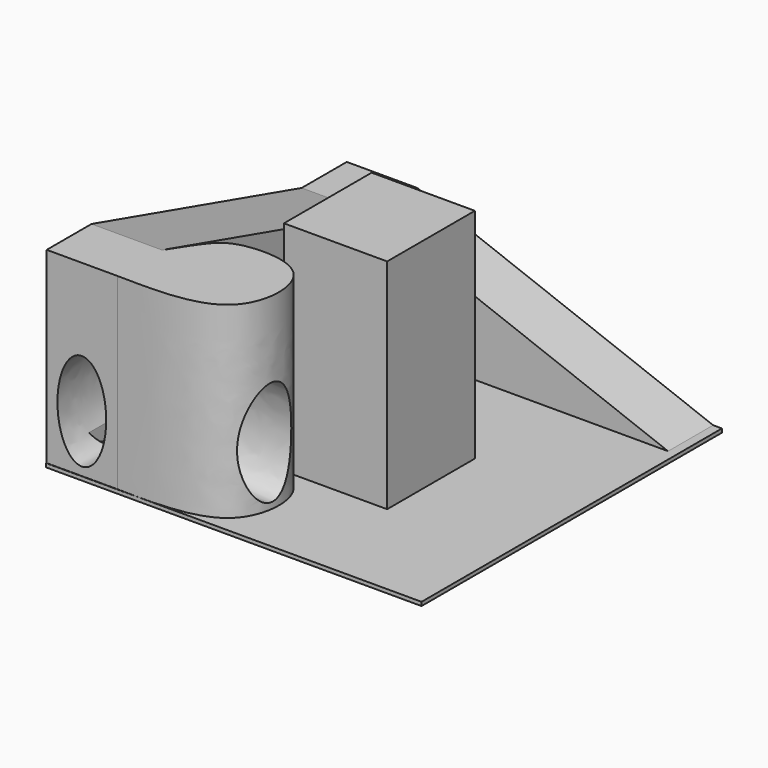
from build123d import *

# Parameters (mm, degrees)
F0_W      = 1000
F0_H      = 1000
F1_DEPTH  = 10
F3_W      = 188.2687941259
F3_H      = 300
F4_DEPTH  = 150
F5_W      = 149.0154206753
F5_H      = 500
F6_DEPTH  = 188
F8_DEPTH  = 500
F12_DEPTH = 453
F14_DEPTH = 800
F16_DEPTH = 133
F17_W     = 274.846598506
F17_H     = 292.0245230198
F18_DEPTH = 581


# Not quite as in the source:
# - the program builds the solid bodies; features that only make, move or delete a surface that nothing else refers to are left out


with BuildPart() as f1:
    # F0 (on Top) → F1 (new body)
    with BuildSketch(Plane.XY):
        Rectangle(F0_W, F0_H)
    extrude(amount=-F1_DEPTH)

    # F3 (on offset) → F4 (join)
    with BuildSketch(Plane.XZ.offset(-500)):
        Polygon((-310.8983501727, 0), (476.5460147594, 0), (-310.8983501727, 300), align=None)
        with Locations((-405.0327472356, 150)):
            Rectangle(F3_W, F3_H)
    extrude(amount=F4_DEPTH)

    # F5 (on face) → F6 (join)
    with BuildSketch(Plane(origin=(-499.1671442986, 0, 0), x_dir=(0, -1, 0), z_dir=(-1, 0, 0))):
        Polygon((350, 500), (-350, 300), (-350, 0), (350, 0), align=None)
        with Locations((424.5077103376, 250)):
            Rectangle(F5_W, F5_H)
    extrude(amount=-F6_DEPTH)

    # F7 (on face) → F8 (join)
    with BuildSketch(Plane.XY.offset(500)):
        with BuildLine():
            Line((-311.1671442986, -350), (-311.1671442986, -499.0154206753))
            add(Edge.make_bspline(
                [(-311.1671442986, -499.0154206753), (-199.0990307789, -500.9048054205), (2.6874525339, -504.3067749137), (10.8332422465, -222.7671703474), (-187.3355186805, -218.6312101857), (-240.2034004178, -248.1285800889), (-268.9803494344, -283.9612428333), (-295.7213113814, -325.8212584641), (-311.1671442986, -350)],
                knots=[0, 0, 0, 0, 0.2545642676, 0.4583607837, 0.6493000717, 0.7654931589, 0.8645466273, 1, 1, 1, 1], degree=3))
        make_face()
    extrude(amount=-F8_DEPTH)

    # F10 (on offset) → F12 (cut)
    with BuildSketch(Plane.YZ.offset(3.8328557014)):
        with BuildLine():
            add(Edge.make_bspline(
                [(-368.5644865036, 16.4244431686), (-238.6606759359, 16.4244431686), (-303.6125812198, 226.7319431686), (-368.5644865036, 437.0394431686), (-433.5163917874, 226.7319431686), (-498.4682970713, 16.4244431686), (-368.5644865036, 16.4244431686)],
                knots=[0, 0, 0, 2.0943951024, 2.0943951024, 4.1887902048, 4.1887902048, 6.2831853072, 6.2831853072, 6.2831853072], degree=2, weights=[1, 0.5, 1, 0.5, 1, 0.5, 1]))
        make_face()
    extrude(amount=-F12_DEPTH, mode=Mode.SUBTRACT)

    # F13 (on face) → F14 (cut)
    with BuildSketch(Plane.XZ.offset(499.0154206753)):
        with BuildLine():
            add(Edge.make_bspline(
                [(-405.5866599083, 22.361529932), (-293.0033574163, 22.361529932), (-349.2950086623, 216.821529932), (-405.5866599083, 411.281529932), (-461.8783111543, 216.821529932), (-518.1699624003, 22.361529932), (-405.5866599083, 22.361529932)],
                knots=[0, 0, 0, 2.0943951024, 2.0943951024, 4.1887902048, 4.1887902048, 6.2831853072, 6.2831853072, 6.2831853072], degree=2, weights=[1, 0.5, 1, 0.5, 1, 0.5, 1]))
        make_face()
    extrude(amount=-F14_DEPTH, mode=Mode.SUBTRACT)

    # F15 (on face) → F16 (cut)
    with BuildSketch(Plane.YZ.offset(-311.1671442986)):
        with BuildLine():
            add(Edge.make_bspline(
                [(248.0068206787, 28.819128871), (356.6426326413, 28.819128871), (302.32472666, 210.5904355645), (248.0068206787, 392.3617422581), (193.6889146974, 210.5904355645), (139.3710087161, 28.819128871), (248.0068206787, 28.819128871)],
                knots=[0, 0, 0, 2.0943951024, 2.0943951024, 4.1887902048, 4.1887902048, 6.2831853072, 6.2831853072, 6.2831853072], degree=2, weights=[1, 0.5, 1, 0.5, 1, 0.5, 1]))
        make_face()
    extrude(amount=-F16_DEPTH, mode=Mode.SUBTRACT)

    # F17 (on face) → F18 (join)
    with BuildSketch(Plane.XY):
        with Locations((46.1656376719, -73.0061382055)):
            Rectangle(F17_W, F17_H)
    extrude(amount=F18_DEPTH)


solid = f1.part
